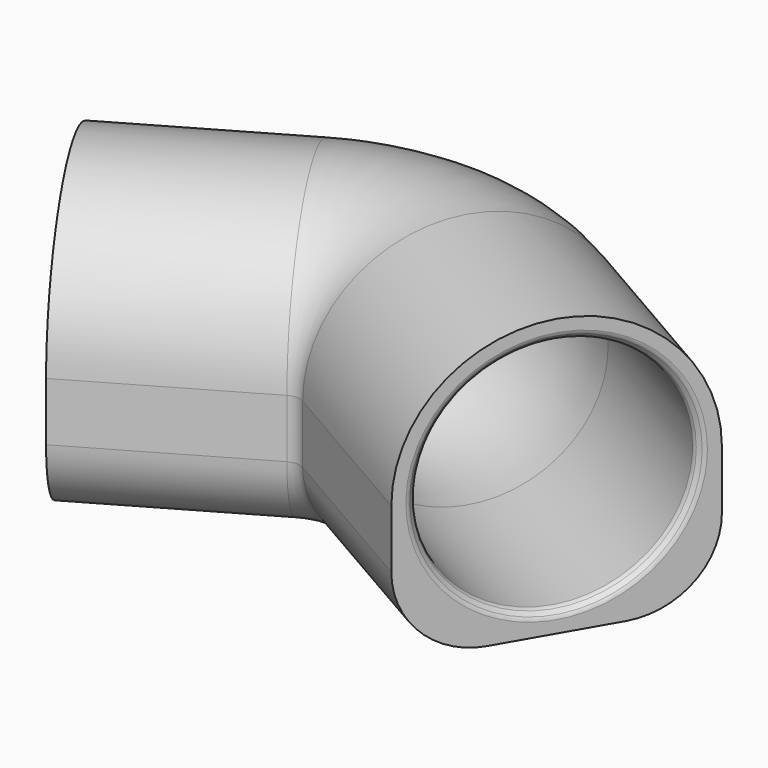
from build123d import *

# Parameters (mm, degrees)
F1_R    = 11.1633
F3_R    = 7.62
F4_SIZE = 0.635
F5_R    = 0.508


with BuildPart() as f2:
    # F2: sweep along a path in F0
    with BuildLine(Plane.XY) as f2_path:
        Line((-21.9970452561, -12.7), (-6.35, -3.6661742094))
        ThreePointArc((-6.35, -3.6661742094), (0, -1.9646968374), (6.35, -3.6661742094))
        Line((6.35, -3.6661742094), (21.9970452561, -12.7))
    # F1 (on Right) → F2 (sweep)
    with BuildSketch(Plane.YZ):
        with BuildLine():
            ThreePointArc((0, -13.1633), (9.3078586928, -9.3078586928), (13.1633, 0))
            ThreePointArc((13.1633, 0), (0, 13.1633), (-13.1633, 0))
            ThreePointArc((-13.1633, 0), (-9.3078586928, -9.3078586928), (0, -13.1633))
        make_face()
        Circle(F1_R, mode=Mode.SUBTRACT)
        with BuildLine():
            Line((13.1633, -13.1633), (13.1633, 0))
            ThreePointArc((13.1633, 0), (9.3078586928, -9.3078586928), (0, -13.1633))
            Line((0, -13.1633), (13.1633, -13.1633))
        make_face()
        with BuildLine():
            ThreePointArc((0, -13.1633), (-9.3078586928, -9.3078586928), (-13.1633, 0))
            Line((-13.1633, 0), (-13.1633, -13.1633))
            Line((-13.1633, -13.1633), (0, -13.1633))
        make_face()
    sweep(path=f2_path.line)

    # F3
    f3_edges = [f2.edges().sort_by_distance(p)[0] for p in [
        (-8.574221, -17.881362, -13.1633),
        (8.574221, -17.881362, -13.1633),
        (0, -13.1633, -13.1633),
        (21.737521, 4.918142, -13.1633),
        (0, 13.1633, -13.1633),
        (-21.737521, 4.918142, -13.1633),
    ]]
    fillet(f3_edges, radius=F3_R)

    # F4
    f4_edges = [f2.edges().sort_by_distance(p)[0] for p in [
        (17.397744, -20.666224, 0),
        (-17.397744, -20.666224, 0),
    ]]
    chamfer(f4_edges, length=F4_SIZE)

    # F5
    f5_edges = [f2.edges().sort_by_distance(p)[0] for p in [
        (-17.080244, -21.21615, 0),
        (-16.847818, -20.348724, 0),
        (17.080244, -21.21615, 0),
        (16.847818, -20.348724, 0),
    ]]
    fillet(f5_edges, radius=F5_R)


solid = f2.part
